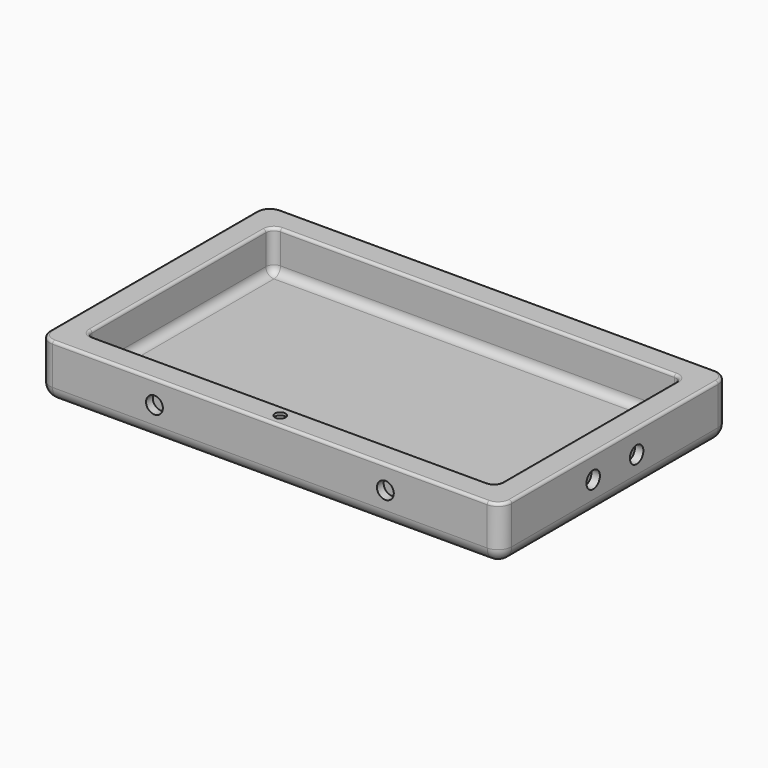
from build123d import *

# Parameters (mm, degrees)
F0_W      = 170
F0_H      = 105
F0_R      = 2
F3_DEPTH  = 20
F4_DEPTH  = 15
F5_R      = 5
F6_R      = 3
F7_R      = 1
F8_R      = 3.1
F9_DEPTH  = 3.1
F10_R     = 3.1
F11_DEPTH = 3.1
F12_R     = 3.1
F13_DEPTH = 3.1
F14_R     = 3.1
F15_DEPTH = 3.1
F16_DEPTH = 1
F17_ANGLE = 180


# Not quite as in the source:
# - a feature names something its author has since deleted; it is built from what else it names


with BuildPart() as f3:
    # F0 (on Top) → F3 (new body)
    with BuildSketch(Plane.XY):
        Rectangle(F0_W, F0_H)
        with Locations((0, -47.75)):
            Circle(F0_R, mode=Mode.SUBTRACT)
        with BuildLine():
            ThreePointArc((-75.5, 40), (-74.6213203436, 42.1213203436), (-72.5, 43))
            Line((-72.5, 43), (72.5, 43))
            ThreePointArc((72.5, 43), (74.6213203436, 42.1213203436), (75.5, 40))
            Line((75.5, 40), (75.5, -40))
            ThreePointArc((75.5, -40), (74.6213203436, -42.1213203436), (72.5, -43))
            Line((72.5, -43), (-72.5, -43))
            ThreePointArc((-72.5, -43), (-74.6213203436, -42.1213203436), (-75.5, -40))
            Line((-75.5, -40), (-75.5, 40))
        make_face(mode=Mode.SUBTRACT)
        with BuildLine():
            Line((72.5, 43), (-72.5, 43))
            ThreePointArc((-72.5, 43), (-74.6213203436, 42.1213203436), (-75.5, 40))
            Line((-75.5, 40), (-75.5, -40))
            ThreePointArc((-75.5, -40), (-74.6213203436, -42.1213203436), (-72.5, -43))
            Line((-72.5, -43), (72.5, -43))
            ThreePointArc((72.5, -43), (74.6213203436, -42.1213203436), (75.5, -40))
            Line((75.5, -40), (75.5, 40))
            ThreePointArc((75.5, 40), (74.6213203436, 42.1213203436), (72.5, 43))
        make_face()
        with Locations((0, -47.75)):
            Circle(F0_R)
    extrude(amount=F3_DEPTH)

    # F0 (on Top) → F4 (cut)
    with BuildSketch(Plane.XY):
        with BuildLine():
            Line((72.5, 43), (-72.5, 43))
            ThreePointArc((-72.5, 43), (-74.6213203436, 42.1213203436), (-75.5, 40))
            Line((-75.5, 40), (-75.5, -40))
            ThreePointArc((-75.5, -40), (-74.6213203436, -42.1213203436), (-72.5, -43))
            Line((-72.5, -43), (72.5, -43))
            ThreePointArc((72.5, -43), (74.6213203436, -42.1213203436), (75.5, -40))
            Line((75.5, -40), (75.5, 40))
            ThreePointArc((75.5, 40), (74.6213203436, 42.1213203436), (72.5, 43))
        make_face()
    extrude(amount=F4_DEPTH, mode=Mode.SUBTRACT)

    # F5
    f5_edges = [f3.edges().sort_by_distance(p)[0] for p in [
        (0, 52.5, 20),
        (-85, 0, 20),
        (0, -52.5, 20),
        (85, 0, 20),
        (85, 52.5, 10),
        (-85, 52.5, 10),
        (-85, -52.5, 10),
        (85, -52.5, 10),
    ]]
    fillet(f5_edges, radius=F5_R)

    # F6
    f6_edges = [f3.edges().sort_by_distance(p)[0] for p in [
        (0, 43, 15),
        (-74.62132, 42.12132, 15),
        (-75.5, 0, 15),
        (-74.62132, -42.12132, 15),
        (0, -43, 15),
        (74.62132, -42.12132, 15),
        (75.5, 0, 15),
        (74.62132, 42.12132, 15),
    ]]
    fillet(f6_edges, radius=F6_R)

    # F7
    f7_edges = [f3.edges().sort_by_distance(p)[0] for p in [
        (0, 52.5, 0),
        (83.535534, 51.035534, 0),
        (-83.535534, 51.035534, 0),
        (85, 0, 0),
        (-85, 0, 0),
        (83.535534, -51.035534, 0),
        (-83.535534, -51.035534, 0),
        (0, -52.5, 0),
        (0, 43, 0),
        (-74.62132, 42.12132, 0),
        (-75.5, 0, 0),
        (-74.62132, -42.12132, 0),
        (0, -43, 0),
        (74.62132, -42.12132, 0),
        (75.5, 0, 0),
        (74.62132, 42.12132, 0),
    ]]
    fillet(f7_edges, radius=F7_R)

    # F8 (on face) → F9 (cut)
    with BuildSketch(Plane.XZ.offset(52.5)):
        with Locations((42.5, 8.5)):
            Circle(F8_R)
        with Locations((-42.5, 8.5)):
            Circle(F8_R)
    extrude(amount=-F9_DEPTH, mode=Mode.SUBTRACT)

    # F10 (on face) → F11 (cut)
    with BuildSketch(Plane(origin=(0, 52.5, 0), x_dir=(-1, 0, 0), z_dir=(0, 1, 0))):
        with Locations((42.5, 8.5)):
            Circle(F10_R)
        with Locations((-42.5, 8.5)):
            Circle(F10_R)
    extrude(amount=-F11_DEPTH, mode=Mode.SUBTRACT)

    # F12 (on face) → F13 (cut)
    with BuildSketch(Plane(origin=(-85, 0, 0), x_dir=(0, -1, 0), z_dir=(-1, 0, 0))):
        with Locations((10, 8.5)):
            Circle(F12_R)
        with Locations((-10, 8.5)):
            Circle(F12_R)
    extrude(amount=-F13_DEPTH, mode=Mode.SUBTRACT)

    # F14 (on face) → F15 (cut)
    with BuildSketch(Plane.YZ.offset(85)):
        with Locations((10, 8.5)):
            Circle(F14_R)
        with Locations((-10, 8.5)):
            Circle(F14_R)
    extrude(amount=-F15_DEPTH, mode=Mode.SUBTRACT)

    # F0 (on Top) → F16 (cut)
    with BuildSketch(Plane.XY):
        with Locations((0, -47.75)):
            Circle(F0_R)
    extrude(amount=F16_DEPTH, mode=Mode.SUBTRACT)


with BuildPart() as f3_1:
    # F17: moved
    add(f3.part.rotate(Axis((0, 0, 0), (0, 1, 0)), F17_ANGLE))


solid = f3_1.part
